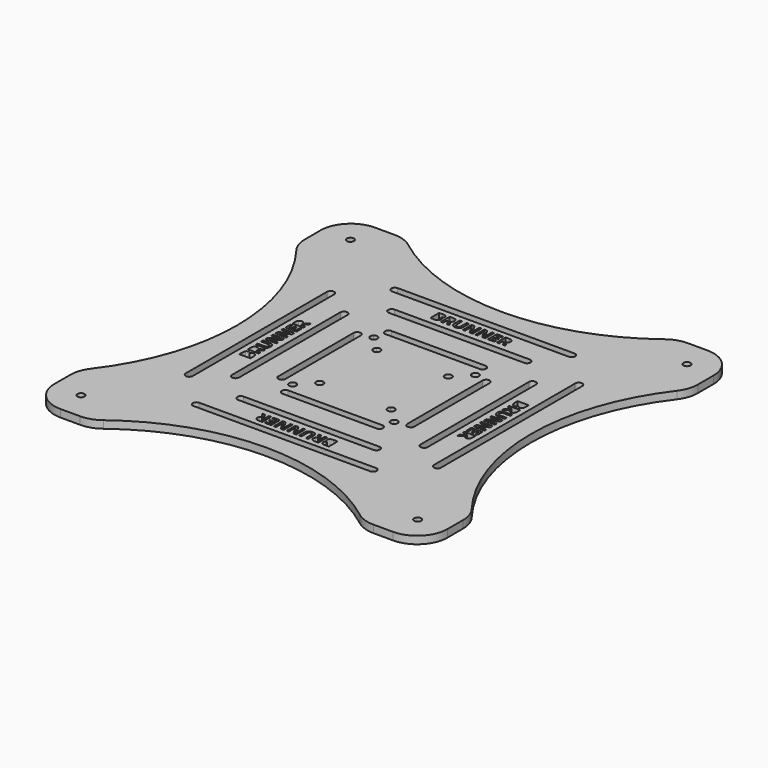
from build123d import *

# Parameters (mm, degrees)
F1_DEPTH = 3.175
F2_COUNT = 4
F2_ANGLE = 270
F3_R     = 12.7


with BuildPart() as f1:
    # F0 (on Top) → F1 (new body)
    with BuildSketch(Plane.XY):
        with BuildLine():
            Line((-57.15, 82.55), (-82.55, 82.55))
            Line((-82.55, 82.55), (-71.7801771252, 71.7801771252))
            ThreePointArc((-71.7801771252, 71.7801771252), (-70.1454918049, 72.1053362522), (-69.2195169534, 70.7195169534))
            ThreePointArc((-69.2195169534, 70.7195169534), (-69.3336976547, 70.1454918049), (-69.6588567816, 69.6588567816))
            Line((-69.6588567816, 69.6588567816), (-22.3887684593, 22.3887684593))
            ThreePointArc((-22.3887684593, 22.3887684593), (-20.754083139, 22.7139275863), (-19.8281082875, 21.3281082875))
            ThreePointArc((-19.8281082875, 21.3281082875), (-19.9422889888, 20.754083139), (-20.2674481158, 20.2674481158))
            Line((-20.2674481158, 20.2674481158), (-16.0606601718, 16.0606601718))
            ThreePointArc((-16.0606601718, 16.0606601718), (-14.4259748515, 16.3858192988), (-13.5, 15))
            ThreePointArc((-13.5, 15), (-13.6141807012, 14.4259748515), (-13.9393398282, 13.9393398282))
            Line((-13.9393398282, 13.9393398282), (0, 0))
            Line((0, 0), (13.9393398282, 13.9393398282))
            ThreePointArc((13.9393398282, 13.9393398282), (13.9393398282, 16.0606601718), (16.0606601718, 16.0606601718))
            Line((16.0606601718, 16.0606601718), (20.2674481158, 20.2674481158))
            ThreePointArc((20.2674481158, 20.2674481158), (20.2674481158, 22.3887684593), (22.3887684593, 22.3887684593))
            Line((22.3887684593, 22.3887684593), (69.6588567816, 69.6588567816))
            ThreePointArc((69.6588567816, 69.6588567816), (69.6588567816, 71.7801771252), (71.7801771252, 71.7801771252))
            Line((71.7801771252, 71.7801771252), (82.55, 82.55))
            Line((82.55, 82.55), (57.15, 82.55))
            ThreePointArc((57.15, 82.55), (0, 61.7461636217), (-57.15, 82.55))
        make_face()
        with BuildLine():
            ThreePointArc((-19.7826923077, 25.575), (-21.2826923077, 27.075), (-19.7826923077, 28.575))
            Line((-19.7826923077, 28.575), (19.7826923077, 28.575))
            ThreePointArc((19.7826923077, 28.575), (21.2826923077, 27.075), (19.7826923077, 25.575))
            Line((19.7826923077, 25.575), (-19.7826923077, 25.575))
        make_face(mode=Mode.SUBTRACT)
        with BuildLine():
            Line((28.4538461538, 38.1), (-28.4538461538, 38.1))
            ThreePointArc((-28.4538461538, 38.1), (-29.9538461538, 39.6), (-28.4538461538, 41.1))
            Line((-28.4538461538, 41.1), (28.4538461538, 41.1))
            ThreePointArc((28.4538461538, 41.1), (29.9538461538, 39.6), (28.4538461538, 38.1))
        make_face(mode=Mode.SUBTRACT)
        with BuildLine():
            Line((-15.5185309995, 43.7277518213), (-15.5185309995, 48.3882072003))
            Line((-15.5185309995, 48.3882072003), (-14.0680675395, 48.3882072003))
            add(Edge.make_bspline(
                [(-14.0680675395, 48.3882072003), (-13.0766115035, 48.3882072003), (-12.6288242609, 48.1061726387)],
                knots=[0, 0, 0, 1, 1, 1], degree=2))
            add(Edge.make_bspline(
                [(-12.6288242609, 48.1061726387), (-12.1810370183, 47.824138077), (-12.1810370183, 47.2090681287)],
                knots=[0, 0, 0, 1, 1, 1], degree=2))
            add(Edge.make_bspline(
                [(-12.1810370183, 47.2090681287), (-12.1810370183, 46.7908613646), (-12.3768801859, 46.5231070339)],
                knots=[0, 0, 0, 1, 1, 1], degree=2))
            add(Edge.make_bspline(
                [(-12.3768801859, 46.5231070339), (-12.5727233535, 46.2553527032), (-12.8981086164, 46.2012918288)],
                knots=[0, 0, 0, 1, 1, 1], degree=2))
            Line((-12.8981086164, 46.2012918288), (-12.8981086164, 46.1696713173))
            add(Edge.make_bspline(
                [(-12.8981086164, 46.1696713173), (-12.4554214563, 46.070729717), (-12.2590682804, 45.7999153368)],
                knots=[0, 0, 0, 1, 1, 1], degree=2))
            add(Edge.make_bspline(
                [(-12.2590682804, 45.7999153368), (-12.0627151045, 45.5291009566), (-12.0627151045, 45.079273681)],
                knots=[0, 0, 0, 1, 1, 1], degree=2))
            add(Edge.make_bspline(
                [(-12.0627151045, 45.079273681), (-12.0627151045, 44.4417633698), (-12.5237625616, 44.0847575956)],
                knots=[0, 0, 0, 1, 1, 1], degree=2))
            add(Edge.make_bspline(
                [(-12.5237625616, 44.0847575956), (-12.9848100187, 43.7277518213), (-13.7753228046, 43.7277518213)],
                knots=[0, 0, 0, 1, 1, 1], degree=2))
            Line((-13.7753228046, 43.7277518213), (-15.5185309995, 43.7277518213))
        make_face(mode=Mode.SUBTRACT)
        with BuildLine():
            Line((-9.6187555755, 45.5158407422), (-10.1440640719, 45.5158407422))
            Line((-10.1440640719, 45.5158407422), (-10.1440640719, 43.7277518213))
            Line((-10.1440640719, 43.7277518213), (-11.1324600584, 43.7277518213))
            Line((-11.1324600584, 43.7277518213), (-11.1324600584, 48.3882072003))
            Line((-11.1324600584, 48.3882072003), (-9.7748180997, 48.3882072003))
            add(Edge.make_bspline(
                [(-9.7748180997, 48.3882072003), (-8.8241627236, 48.3882072003), (-8.3687253573, 48.0424216075)],
                knots=[0, 0, 0, 1, 1, 1], degree=2))
            add(Edge.make_bspline(
                [(-8.3687253573, 48.0424216075), (-7.913287991, 47.6966360147), (-7.913287991, 46.9918046147)],
                knots=[0, 0, 0, 1, 1, 1], degree=2))
            add(Edge.make_bspline(
                [(-7.913287991, 46.9918046147), (-7.913287991, 46.580737966), (-8.1392216453, 46.2604527856)],
                knots=[0, 0, 0, 1, 1, 1], degree=2))
            add(Edge.make_bspline(
                [(-8.1392216453, 46.2604527856), (-8.3651552995, 45.9401676053), (-8.7803020142, 45.7586046687)],
                knots=[0, 0, 0, 1, 1, 1], degree=2))
            add(Edge.make_bspline(
                [(-8.7803020142, 45.7586046687), (-7.7276449883, 44.1867592453), (-7.409399841, 43.7277518213)],
                knots=[0, 0, 0, 1, 1, 1], degree=2))
            Line((-7.409399841, 43.7277518213), (-8.5059175763, 43.7277518213))
            Line((-8.5059175763, 43.7277518213), (-9.6187555755, 45.5158407422))
        make_face(mode=Mode.SUBTRACT)
        with BuildLine():
            Line((-4.0147849359, 48.3882072003), (-3.0294489989, 48.3882072003))
            Line((-3.0294489989, 48.3882072003), (-3.0294489989, 45.3730384324))
            add(Edge.make_bspline(
                [(-3.0294489989, 45.3730384324), (-3.0294489989, 44.855890068), (-3.2604827356, 44.4672637823)],
                knots=[0, 0, 0, 1, 1, 1], degree=2))
            add(Edge.make_bspline(
                [(-3.2604827356, 44.4672637823), (-3.4915164724, 44.0786374966), (-3.9285935418, 43.8710641392)],
                knots=[0, 0, 0, 1, 1, 1], degree=2))
            add(Edge.make_bspline(
                [(-3.9285935418, 43.8710641392), (-4.3656706112, 43.6634907819), (-4.9613602459, 43.6634907819)],
                knots=[0, 0, 0, 1, 1, 1], degree=2))
            add(Edge.make_bspline(
                [(-4.9613602459, 43.6634907819), (-5.8599947806, 43.6634907819), (-6.3572528234, 44.124538239)],
                knots=[0, 0, 0, 1, 1, 1], degree=2))
            add(Edge.make_bspline(
                [(-6.3572528234, 44.124538239), (-6.8545108661, 44.585585696), (-6.8545108661, 45.3852786304)],
                knots=[0, 0, 0, 1, 1, 1], degree=2))
            Line((-6.8545108661, 45.3852786304), (-6.8545108661, 48.3882072003))
            Line((-6.8545108661, 48.3882072003), (-5.8701949456, 48.3882072003))
            Line((-5.8701949456, 48.3882072003), (-5.8701949456, 45.5352210556))
            add(Edge.make_bspline(
                [(-5.8701949456, 45.5352210556), (-5.8701949456, 44.9966523447), (-5.6534414398, 44.7447082697)],
                knots=[0, 0, 0, 1, 1, 1], degree=2))
            add(Edge.make_bspline(
                [(-5.6534414398, 44.7447082697), (-5.436687934, 44.4927641947), (-4.9358598335, 44.4927641947)],
                knots=[0, 0, 0, 1, 1, 1], degree=2))
            add(Edge.make_bspline(
                [(-4.9358598335, 44.4927641947), (-4.451351997, 44.4927641947), (-4.2330684664, 44.7462382945)],
                knots=[0, 0, 0, 1, 1, 1], degree=2))
            add(Edge.make_bspline(
                [(-4.2330684664, 44.7462382945), (-4.0147849359, 44.9997123942), (-4.0147849359, 45.5413411546)],
                knots=[0, 0, 0, 1, 1, 1], degree=2))
            Line((-4.0147849359, 45.5413411546), (-4.0147849359, 48.3882072003))
        make_face(mode=Mode.SUBTRACT)
        with BuildLine():
            Line((37.125, 50.625), (-37.125, 50.625))
            ThreePointArc((-37.125, 50.625), (-38.625, 52.125), (-37.125, 53.625))
            Line((-37.125, 53.625), (37.125, 53.625))
            ThreePointArc((37.125, 53.625), (38.625, 52.125), (37.125, 50.625))
        make_face(mode=Mode.SUBTRACT)
        with BuildLine():
            Line((2.2460763284, 48.3882072003), (2.2460763284, 43.7277518213))
            Line((2.2460763284, 43.7277518213), (0.9904360195, 43.7277518213))
            Line((0.9904360195, 43.7277518213), (-1.0373567784, 47.2529288381))
            Line((-1.0373567784, 47.2529288381), (-1.0659172403, 47.2529288381))
            add(Edge.make_bspline(
                [(-1.0659172403, 47.2529288381), (-1.0047162505, 46.3196137425), (-1.0047162505, 45.9207872918)],
                knots=[0, 0, 0, 1, 1, 1], degree=2))
            Line((-1.0047162505, 45.9207872918), (-1.0047162505, 43.7277518213))
            Line((-1.0047162505, 43.7277518213), (-1.8880505377, 43.7277518213))
            Line((-1.8880505377, 43.7277518213), (-1.8880505377, 48.3882072003))
            Line((-1.8880505377, 48.3882072003), (-0.6415903772, 48.3882072003))
            Line((-0.6415903772, 48.3882072003), (1.3821223547, 44.8977107444))
            Line((1.3821223547, 44.8977107444), (1.4045627177, 44.8977107444))
            add(Edge.make_bspline(
                [(1.4045627177, 44.8977107444), (1.3566219423, 45.8065454441), (1.3566219423, 46.1819115153)],
                knots=[0, 0, 0, 1, 1, 1], degree=2))
            Line((1.3566219423, 46.1819115153), (1.3566219423, 48.3882072003))
            Line((1.3566219423, 48.3882072003), (2.2460763284, 48.3882072003))
        make_face(mode=Mode.SUBTRACT)
        with BuildLine():
            Line((7.5532221672, 48.3882072003), (7.5532221672, 43.7277518213))
            Line((7.5532221672, 43.7277518213), (6.2975818582, 43.7277518213))
            Line((6.2975818582, 43.7277518213), (4.2697890603, 47.2529288381))
            Line((4.2697890603, 47.2529288381), (4.2412285984, 47.2529288381))
            add(Edge.make_bspline(
                [(4.2412285984, 47.2529288381), (4.3024295883, 46.3196137425), (4.3024295883, 45.9207872918)],
                knots=[0, 0, 0, 1, 1, 1], degree=2))
            Line((4.3024295883, 45.9207872918), (4.3024295883, 43.7277518213))
            Line((4.3024295883, 43.7277518213), (3.4190953011, 43.7277518213))
            Line((3.4190953011, 43.7277518213), (3.4190953011, 48.3882072003))
            Line((3.4190953011, 48.3882072003), (4.6655554615, 48.3882072003))
            Line((4.6655554615, 48.3882072003), (6.6892681934, 44.8977107444))
            Line((6.6892681934, 44.8977107444), (6.7117085564, 44.8977107444))
            add(Edge.make_bspline(
                [(6.7117085564, 44.8977107444), (6.663767781, 45.8065454441), (6.663767781, 46.1819115153)],
                knots=[0, 0, 0, 1, 1, 1], degree=2))
            Line((6.663767781, 46.1819115153), (6.663767781, 48.3882072003))
            Line((6.663767781, 48.3882072003), (7.5532221672, 48.3882072003))
        make_face(mode=Mode.SUBTRACT)
        Polygon((11.4099045459, 44.5437650196), (11.4099045459, 43.7277518213), (8.7262411398, 43.7277518213), (8.7262411398, 48.3882072003), (11.4099045459, 48.3882072003), (11.4099045459, 47.578314101), (9.7146371263, 47.578314101), (9.7146371263, 46.5552375535), (11.2926026486, 46.5552375535), (11.2926026486, 45.7453444542), (9.7146371263, 45.7453444542), (9.7146371263, 44.5437650196), align=None, mode=Mode.SUBTRACT)
        with BuildLine():
            Line((13.8956847513, 45.5158407422), (13.3703762549, 45.5158407422))
            Line((13.3703762549, 45.5158407422), (13.3703762549, 43.7277518213))
            Line((13.3703762549, 43.7277518213), (12.3819802684, 43.7277518213))
            Line((12.3819802684, 43.7277518213), (12.3819802684, 48.3882072003))
            Line((12.3819802684, 48.3882072003), (13.7396222271, 48.3882072003))
            add(Edge.make_bspline(
                [(13.7396222271, 48.3882072003), (14.6902776032, 48.3882072003), (15.1457149695, 48.0424216075)],
                knots=[0, 0, 0, 1, 1, 1], degree=2))
            add(Edge.make_bspline(
                [(15.1457149695, 48.0424216075), (15.6011523359, 47.6966360147), (15.6011523359, 46.9918046147)],
                knots=[0, 0, 0, 1, 1, 1], degree=2))
            add(Edge.make_bspline(
                [(15.6011523359, 46.9918046147), (15.6011523359, 46.580737966), (15.3752186816, 46.2604527856)],
                knots=[0, 0, 0, 1, 1, 1], degree=2))
            add(Edge.make_bspline(
                [(15.3752186816, 46.2604527856), (15.1492850273, 45.9401676053), (14.7341383126, 45.7586046687)],
                knots=[0, 0, 0, 1, 1, 1], degree=2))
            add(Edge.make_bspline(
                [(14.7341383126, 45.7586046687), (15.7867953385, 44.1867592453), (16.1050404859, 43.7277518213)],
                knots=[0, 0, 0, 1, 1, 1], degree=2))
            Line((16.1050404859, 43.7277518213), (15.0085227506, 43.7277518213))
            Line((15.0085227506, 43.7277518213), (13.8956847513, 45.5158407422))
        make_face(mode=Mode.SUBTRACT)
    extrude(amount=F1_DEPTH)

    # F2: F1 ×4 about axis
    f2_axis = Axis((0, 0, 1.5875), (0, 0, -1))


with BuildPart() as f1_1:
    add(f1.part)
    for i in range(1, F2_COUNT):
        add(f1.part.rotate(f2_axis, i * F2_ANGLE / (F2_COUNT - 1)))

    # F3
    f3_edges = [f1_1.edges().sort_by_distance(p)[0] for p in [
        (-82.55, 82.55, 1.5875),
        (82.55, 82.55, 1.5875),
        (82.55, -82.55, 1.5875),
        (-82.55, -82.55, 1.5875),
        (-57.15, -82.55, 1.5875),
        (57.15, -82.55, 1.5875),
        (-82.55, -57.15, 1.5875),
        (-82.55, 57.15, 1.5875),
        (-57.15, 82.55, 1.5875),
        (82.55, -57.15, 1.5875),
        (82.55, 57.15, 1.5875),
        (57.15, 82.55, 1.5875),
    ]]
    fillet(f3_edges, radius=F3_R)


solid = f1_1.part
